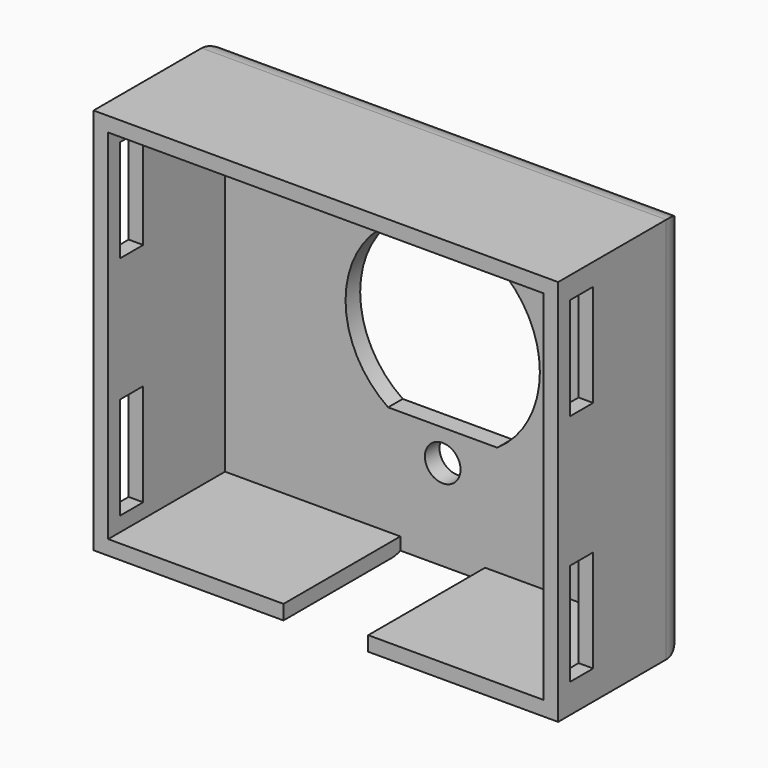
from build123d import *

# Parameters (mm, degrees)
F0_W         = 80.772
F0_H         = 67.3239192
F0_R         = 3.0975808
F1_DEPTH     = 3.175
F2_W         = 80.772
F2_H         = 67.3239192
F2_W_2       = 75.692
F2_H_2       = 62.2439192
F3_DEPTH     = 25.4
F4_W         = 14.732
F4_H         = 25.4
F5_DEPTH     = 25.4
F6_W         = 5.08
F6_H         = 17.78
F7_DEPTH     = 25.4
F8_W         = 5.08
F8_H         = 17.78
F9_DEPTH     = 25.4
F10_T1_DEPTH = 106.172
F10_T3_DEPTH = 92.7239192


# Not quite as in the source:
# - a fillet or chamfer that OpenCascade refuses, or shapes differently, is made with other operations: its cross-section is extruded or revolved along the edge and cut away or added


with BuildPart() as f1:
    # F0 (on Front) → F1 (new body)
    with BuildSketch(Plane.XZ):
        Rectangle(F0_W, F0_H)
        with Locations((0, -17.5051212)):
            Circle(F0_R, mode=Mode.SUBTRACT)
        with BuildLine():
            Line((9.4944692, -12.0580404), (-9.4944692, -12.0580404))
            ThreePointArc((-9.4944692, -12.0580404), (-16.8909981247, 1.9119596), (-9.4944692, 15.8819596))
            Line((-9.4944692, 15.8819596), (9.4944692, 15.8819596))
            ThreePointArc((9.4944692, 15.8819596), (16.8909981247, 1.9119596), (9.4944692, -12.0580404))
        make_face(mode=Mode.SUBTRACT)
    extrude(amount=F1_DEPTH)

    # F2 (on face) → F3 (join)
    with BuildSketch(Plane.XZ.offset(3.175)):
        Rectangle(F2_W, F2_H)
        Rectangle(F2_W_2, F2_H_2, mode=Mode.SUBTRACT)
    extrude(amount=F3_DEPTH)

    # F4 (on face) → F5 (cut)
    with BuildSketch(Plane.XY.offset(-31.1219596)):
        with Locations((0, -15.875)):
            Rectangle(F4_W, F4_H)
    extrude(amount=-F5_DEPTH, mode=Mode.SUBTRACT)

    # F6 (on face) → F7 (cut)
    with BuildSketch(Plane.YZ.offset(40.386)):
        with Locations((-23.495, 20.9619596)):
            Rectangle(F6_W, F6_H)
        with Locations((-23.495, -19.6919596)):
            Rectangle(F6_W, F6_H)
    extrude(amount=-F7_DEPTH, mode=Mode.SUBTRACT)

    # F8 (on face) → F9 (cut)
    with BuildSketch(Plane(origin=(-40.386, 0, 0), x_dir=(0, -1, 0), z_dir=(-1, 0, 0))):
        with Locations((23.495, 19.6919596)):
            Rectangle(F8_W, F8_H)
        with Locations((23.495, -19.6919596)):
            Rectangle(F8_W, F8_H)
    extrude(amount=-F9_DEPTH, mode=Mode.SUBTRACT)

    # F10: fillet of radius 5.08 on 4 edges, made by hand

    # F10_s2 → F10_t1 (cut)
    with BuildSketch(Plane.YZ.offset(-53.086)):
        with BuildLine():
            ThreePointArc((0, 28.5819596), (-1.4878975516, 32.1740620484), (-5.08, 33.6619596))
            Line((-5.08, 33.6619596), (0, 33.6619596))
            Line((0, 33.6619596), (0, 28.5819596))
        make_face()
        with BuildLine():
            ThreePointArc((-5.08, -33.6619596), (-1.4878975516, -32.1740620484), (0, -28.5819596))
            Line((0, -28.5819596), (0, -33.6619596))
            Line((0, -33.6619596), (-5.08, -33.6619596))
        make_face()
    extrude(amount=F10_T1_DEPTH, mode=Mode.SUBTRACT)

    # F10_s4 → F10_t3 (cut)
    with BuildSketch(Plane.XY.offset(-46.3619596)):
        with BuildLine():
            ThreePointArc((-35.306, 0), (-38.8981024484, -1.4878975516), (-40.386, -5.08))
            Line((-40.386, -5.08), (-40.386, 0))
            Line((-40.386, 0), (-35.306, 0))
        make_face()
        with BuildLine():
            ThreePointArc((40.386, -5.08), (38.8981024484, -1.4878975516), (35.306, 0))
            Line((35.306, 0), (40.386, 0))
            Line((40.386, 0), (40.386, -5.08))
        make_face()
    extrude(amount=F10_T3_DEPTH, mode=Mode.SUBTRACT)


solid = f1.part
